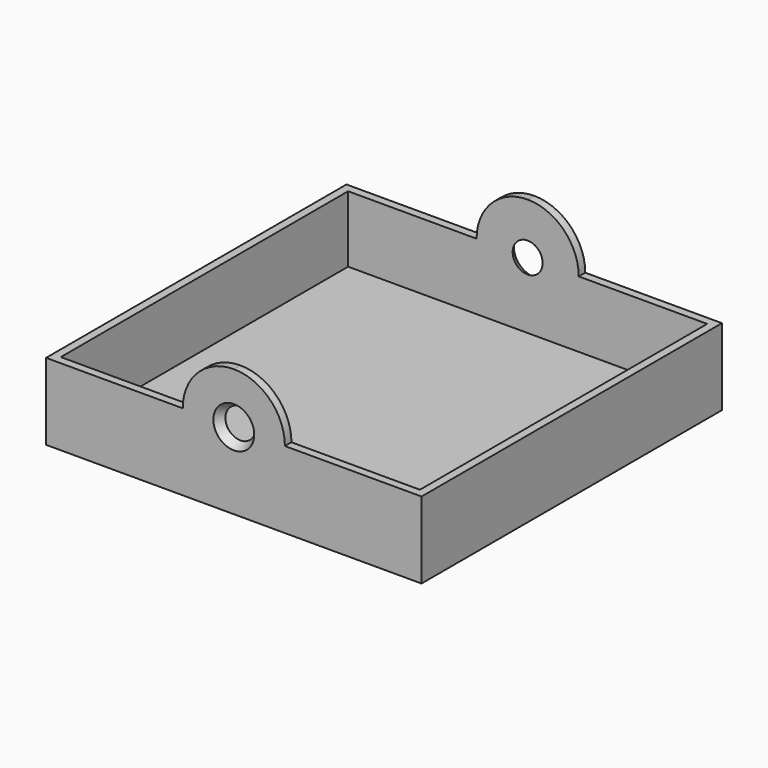
from build123d import *

# Parameters (mm, degrees)
F1_DEPTH = 73.5
F2_W     = 70.3
F2_H     = 70.3
F3_DEPTH = 23
F4_DEPTH = 73.501


# Not quite as in the source:
# - a fillet or chamfer that OpenCascade refuses, or shapes differently, is made with other operations: its cross-section is extruded or revolved along the edge and cut away or added


with BuildPart() as f1:
    # F0 (on Front) → F1 (new body)
    with BuildSketch(Plane.XZ):
        with BuildLine():
            Line((0, 15), (0, 0))
            Line((0, 0), (73.5, 0))
            Line((73.5, 0), (73.5, 15))
            Line((73.5, 15), (46.75, 15))
            Line((46.75, 15), (38.75, 15))
            ThreePointArc((38.75, 15), (36.75, 13), (34.75, 15))
            Line((34.75, 15), (26.75, 15))
            Line((26.75, 15), (0, 15))
        make_face()
        with BuildLine():
            Line((0, 25), (0, 15))
            Line((0, 15), (26.75, 15))
            ThreePointArc((26.75, 15), (29.6789321881, 22.0710678119), (36.75, 25))
            Line((36.75, 25), (0, 25))
        make_face()
        with BuildLine():
            Line((46.75, 15), (73.5, 15))
            Line((73.5, 15), (73.5, 25))
            Line((73.5, 25), (36.75, 25))
            ThreePointArc((36.75, 25), (43.8210678119, 22.0710678119), (46.75, 15))
        make_face()
        with BuildLine():
            ThreePointArc((36.75, 25), (29.6789321881, 22.0710678119), (26.75, 15))
            Line((26.75, 15), (34.75, 15))
            ThreePointArc((34.75, 15), (36.75, 17), (38.75, 15))
            Line((38.75, 15), (46.75, 15))
            ThreePointArc((46.75, 15), (43.8210678119, 22.0710678119), (36.75, 25))
        make_face()
    extrude(amount=-F1_DEPTH)

    # F2 (on face) → F3 (cut)
    with BuildSketch(Plane.XY.offset(25)):
        with Locations((36.75, 36.75)):
            Rectangle(F2_W, F2_H)
    extrude(amount=-F3_DEPTH, mode=Mode.SUBTRACT)

    # F0 (on Front) → F4 (cut, through all)
    with BuildSketch(Plane.XZ):
        with BuildLine():
            Line((0, 25), (0, 15))
            Line((0, 15), (26.75, 15))
            ThreePointArc((26.75, 15), (29.6789321881, 22.0710678119), (36.75, 25))
            Line((36.75, 25), (0, 25))
        make_face()
        with BuildLine():
            Line((46.75, 15), (73.5, 15))
            Line((73.5, 15), (73.5, 25))
            Line((73.5, 25), (36.75, 25))
            ThreePointArc((36.75, 25), (43.8210678119, 22.0710678119), (46.75, 15))
        make_face()
    extrude(amount=-F4_DEPTH, mode=Mode.SUBTRACT)

    # F5: chamfer of 3 x 2 on 1 edges, made by hand

    # F5_s1 → F5_t2 (revolve, cut)
    with BuildSketch(Plane.XY.offset(15)):
        Polygon((34.75, 3), (32.75, 0), (34.75, 0), align=None)
    revolve(axis=Axis((36.75, 0, 15), (0, 1, 0)), mode=Mode.SUBTRACT)

    # F6: chamfer of 3 x 2 on 1 edges, made by hand

    # F6_s1 → F6_t2 (revolve, cut)
    with BuildSketch(Plane.XY.offset(15)):
        Polygon((32.75, 73.5), (34.75, 70.5), (34.75, 73.5), align=None)
    revolve(axis=Axis((36.75, 73.5, 15), (0, 1, 0)), mode=Mode.SUBTRACT)


solid = f1.part
